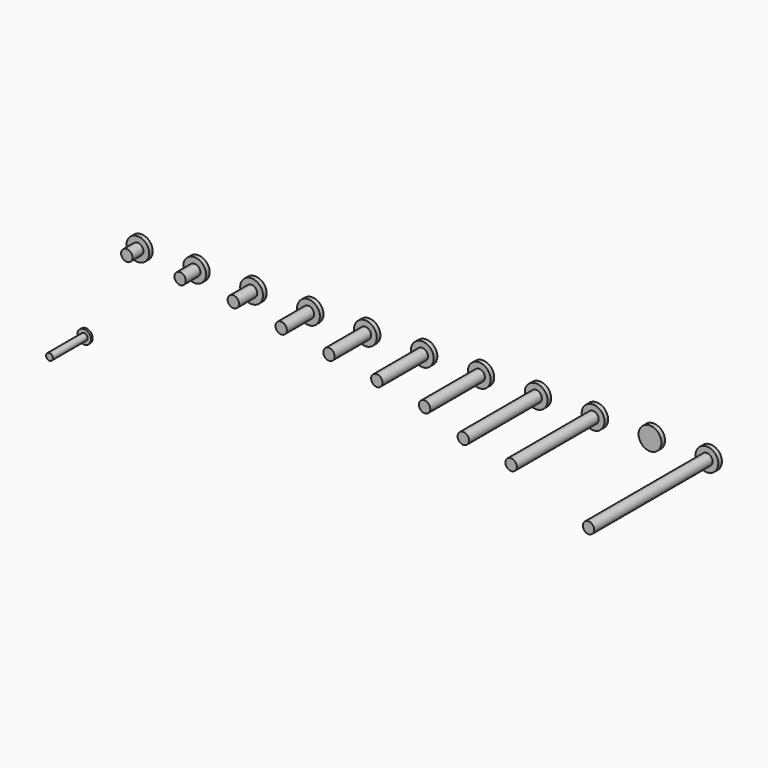
from build123d import *

# Parameters (mm, degrees)
F0_R      = 5
F0_R_2    = 2.5
F1_DEPTH  = 2
F2_DEPTH  = 6
F3_DEPTH  = 8
F4_DEPTH  = 10
F5_DEPTH  = 15
F6_DEPTH  = 20
F7_DEPTH  = 25
F8_DEPTH  = 30
F9_DEPTH  = 40
F10_DEPTH = 45
F12_DEPTH = 65
F0_R_3    = 3
F0_R_4    = 1.5
F13_DEPTH = 1
F14_DEPTH = 20


# Not quite as in the source:
# - the program builds the solid bodies; features that only make, move or delete a surface that nothing else refers to are left out


with BuildPart() as f1:
    # F0 (on Front) → F1 (new body)
    with BuildSketch(Plane.XZ):
        with Locations((-18.9229398966, -7.2633498348)):
            Circle(F0_R)
        with Locations((-18.9229398966, -7.2633498348)):
            Circle(F0_R_2, mode=Mode.SUBTRACT)
        with Locations((-18.9229398966, -7.2633498348)):
            Circle(F0_R_2)
    extrude(amount=-F1_DEPTH)

    # F0 (on Front) → F2 (join)
    with BuildSketch(Plane.XZ):
        with Locations((-18.9229398966, -7.2633498348)):
            Circle(F0_R_2)
    extrude(amount=F2_DEPTH)


with BuildPart() as f1b:
    # F0 (on Front) → F1, piece 2 (new body)
    with BuildSketch(Plane.XZ):
        with Locations((6.0770601034, -7.2633498348)):
            Circle(F0_R)
        with Locations((6.0770601034, -7.2633498348)):
            Circle(F0_R_2, mode=Mode.SUBTRACT)
        with Locations((6.0770601034, -7.2633498348)):
            Circle(F0_R_2)
    extrude(amount=-F1_DEPTH)

    # F0 (on Front) → F3 (join)
    with BuildSketch(Plane.XZ):
        with Locations((6.0770601034, -7.2633498348)):
            Circle(F0_R_2)
    extrude(amount=F3_DEPTH)


with BuildPart() as f1c:
    # F0 (on Front) → F1, piece 3 (new body)
    with BuildSketch(Plane.XZ):
        with Locations((31.0770601034, -7.2633498348)):
            Circle(F0_R)
        with Locations((31.0770601034, -7.2633498348)):
            Circle(F0_R_2, mode=Mode.SUBTRACT)
        with Locations((31.0770601034, -7.2633498348)):
            Circle(F0_R_2)
    extrude(amount=-F1_DEPTH)

    # F0 (on Front) → F4 (join)
    with BuildSketch(Plane.XZ):
        with Locations((31.0770601034, -7.2633498348)):
            Circle(F0_R_2)
    extrude(amount=F4_DEPTH)


with BuildPart() as f1d:
    # F0 (on Front) → F1, piece 4 (new body)
    with BuildSketch(Plane.XZ):
        with Locations((56.0770601034, -7.2633498348)):
            Circle(F0_R)
        with Locations((56.0770601034, -7.2633498348)):
            Circle(F0_R_2, mode=Mode.SUBTRACT)
        with Locations((56.0770601034, -7.2633498348)):
            Circle(F0_R_2)
    extrude(amount=-F1_DEPTH)

    # F0 (on Front) → F5 (join)
    with BuildSketch(Plane.XZ):
        with Locations((56.0770601034, -7.2633498348)):
            Circle(F0_R_2)
    extrude(amount=F5_DEPTH)


with BuildPart() as f1e:
    # F0 (on Front) → F1, piece 5 (new body)
    with BuildSketch(Plane.XZ):
        with Locations((156.0770601034, -7.2633498348)):
            Circle(F0_R)
        with Locations((156.0770601034, -7.2633498348)):
            Circle(F0_R_2, mode=Mode.SUBTRACT)
        with Locations((156.0770601034, -7.2633498348)):
            Circle(F0_R_2)
    extrude(amount=-F1_DEPTH)

    # F0 (on Front) → F9 (join)
    with BuildSketch(Plane.XZ):
        with Locations((156.0770601034, -7.2633498348)):
            Circle(F0_R_2)
    extrude(amount=F9_DEPTH)


with BuildPart() as f1f:
    # F0 (on Front) → F1, piece 6 (new body)
    with BuildSketch(Plane.XZ):
        with Locations((131.0770601034, -7.2633498348)):
            Circle(F0_R)
        with Locations((131.0770601034, -7.2633498348)):
            Circle(F0_R_2, mode=Mode.SUBTRACT)
        with Locations((131.0770601034, -7.2633498348)):
            Circle(F0_R_2)
    extrude(amount=-F1_DEPTH)

    # F0 (on Front) → F8 (join)
    with BuildSketch(Plane.XZ):
        with Locations((131.0770601034, -7.2633498348)):
            Circle(F0_R_2)
    extrude(amount=F8_DEPTH)


with BuildPart() as f1g:
    # F0 (on Front) → F1, piece 7 (new body)
    with BuildSketch(Plane.XZ):
        with Locations((106.0770601034, -7.2633498348)):
            Circle(F0_R)
        with Locations((106.0770601034, -7.2633498348)):
            Circle(F0_R_2, mode=Mode.SUBTRACT)
        with Locations((106.0770601034, -7.2633498348)):
            Circle(F0_R_2)
    extrude(amount=-F1_DEPTH)

    # F0 (on Front) → F7 (join)
    with BuildSketch(Plane.XZ):
        with Locations((106.0770601034, -7.2633498348)):
            Circle(F0_R_2)
    extrude(amount=F7_DEPTH)


with BuildPart() as f1h:
    # F0 (on Front) → F1, piece 8 (new body)
    with BuildSketch(Plane.XZ):
        with Locations((81.0770601034, -7.2633498348)):
            Circle(F0_R)
        with Locations((81.0770601034, -7.2633498348)):
            Circle(F0_R_2, mode=Mode.SUBTRACT)
        with Locations((81.0770601034, -7.2633498348)):
            Circle(F0_R_2)
    extrude(amount=-F1_DEPTH)

    # F0 (on Front) → F6 (join)
    with BuildSketch(Plane.XZ):
        with Locations((81.0770601034, -7.2633498348)):
            Circle(F0_R_2)
    extrude(amount=F6_DEPTH)


with BuildPart() as f1i:
    # F0 (on Front) → F1, piece 9 (new body)
    with BuildSketch(Plane.XZ):
        with Locations((206.0770601034, -7.2633498348)):
            Circle(F0_R)
        with Locations((206.0770601034, -7.2633498348)):
            Circle(F0_R_2, mode=Mode.SUBTRACT)
        with Locations((206.0770601034, -7.2633498348)):
            Circle(F0_R_2)
    extrude(amount=-F1_DEPTH)


with BuildPart() as f1j:
    # F0 (on Front) → F1, piece 10 (new body)
    with BuildSketch(Plane.XZ):
        with Locations((181.0770601034, -7.2633498348)):
            Circle(F0_R)
        with Locations((181.0770601034, -7.2633498348)):
            Circle(F0_R_2, mode=Mode.SUBTRACT)
        with Locations((181.0770601034, -7.2633498348)):
            Circle(F0_R_2)
    extrude(amount=-F1_DEPTH)

    # F0 (on Front) → F10 (join)
    with BuildSketch(Plane.XZ):
        with Locations((181.0770601034, -7.2633498348)):
            Circle(F0_R_2)
    extrude(amount=F10_DEPTH)


with BuildPart() as f1k:
    # F0 (on Front) → F1, piece 11 (new body)
    with BuildSketch(Plane.XZ):
        with Locations((231.0770601034, -7.2633498348)):
            Circle(F0_R)
        with Locations((231.0770601034, -7.2633498348)):
            Circle(F0_R_2, mode=Mode.SUBTRACT)
        with Locations((231.0770601034, -7.2633498348)):
            Circle(F0_R_2)
    extrude(amount=-F1_DEPTH)

    # F0 (on Front) → F12 (join)
    with BuildSketch(Plane.XZ):
        with Locations((231.0770601034, -7.2633498348)):
            Circle(F0_R_2)
    extrude(amount=F12_DEPTH)


with BuildPart() as f13:
    # F0 (on Front) → F13 (new body)
    with BuildSketch(Plane.XZ):
        with Locations((-41.6826158762, -48.1766760349)):
            Circle(F0_R_3)
        with Locations((-41.6826158762, -48.1766760349)):
            Circle(F0_R_4, mode=Mode.SUBTRACT)
    extrude(amount=F13_DEPTH)

    # F0 (on Front) → F14 (join)
    with BuildSketch(Plane.XZ):
        with Locations((-41.6826158762, -48.1766760349)):
            Circle(F0_R_4)
    extrude(amount=F14_DEPTH)


solid = Compound([f1.part, f1b.part, f1c.part, f1d.part, f1e.part, f1f.part, f1g.part, f1h.part, f1i.part, f1j.part, f1k.part, f13.part])
